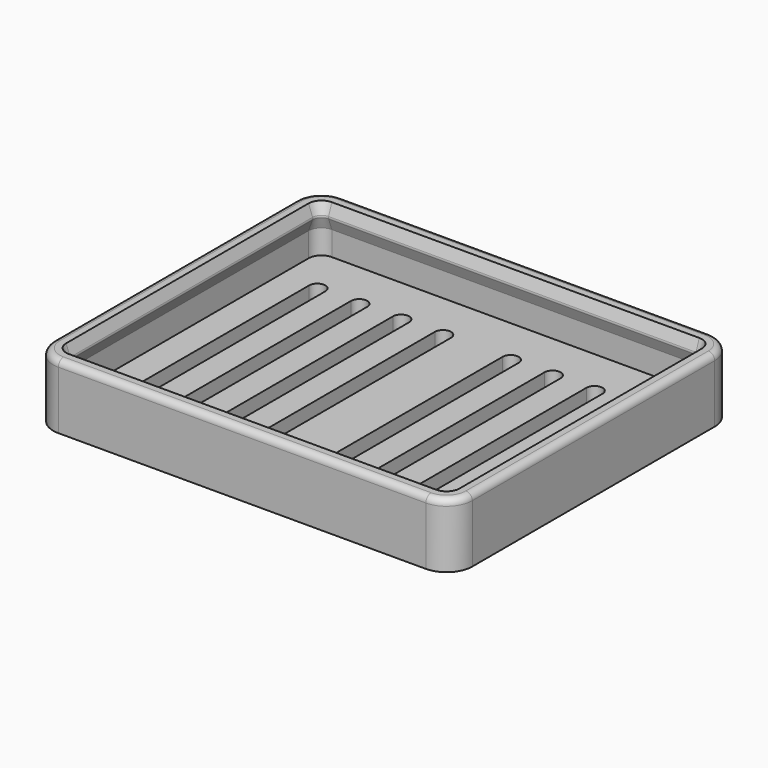
from build123d import *

# Parameters (mm, degrees)
F0_W     = 65
F0_H     = 55
F0_W_2   = 61
F0_H_2   = 51
F1_DEPTH = 2.5
F2_DEPTH = 10
F3_R     = 2
F4_R     = 4
F7_R     = 1


with BuildPart() as f1:
    # F0 (on Top) → F1 (new body)
    with BuildSketch(Plane.XY):
        Rectangle(F0_W, F0_H)
        Rectangle(F0_W_2, F0_H_2, mode=Mode.SUBTRACT)
        Rectangle(F0_W_2, F0_H_2)
        with BuildLine():
            ThreePointArc((-26, 18), (-24.75, 19.25), (-23.5, 18))
            Line((-23.5, 18), (-23.5, -18))
            ThreePointArc((-23.5, -18), (-24.75, -19.25), (-26, -18))
            Line((-26, -18), (-26, 18))
        make_face(mode=Mode.SUBTRACT)
        with BuildLine():
            Line((-19.5, -18), (-19.5, 18))
            ThreePointArc((-19.5, 18), (-18.25, 19.25), (-17, 18))
            Line((-17, 18), (-17, -18))
            ThreePointArc((-17, -18), (-18.25, -19.25), (-19.5, -18))
        make_face(mode=Mode.SUBTRACT)
        with BuildLine():
            Line((-13, -18), (-13, 18))
            ThreePointArc((-13, 18), (-11.75, 19.25), (-10.5, 18))
            Line((-10.5, 18), (-10.5, -18))
            ThreePointArc((-10.5, -18), (-11.75, -19.25), (-13, -18))
        make_face(mode=Mode.SUBTRACT)
        with BuildLine():
            Line((-6.5, -18), (-6.5, 18))
            ThreePointArc((-6.5, 18), (-5.25, 19.25), (-4, 18))
            Line((-4, 18), (-4, -18))
            ThreePointArc((-4, -18), (-5.25, -19.25), (-6.5, -18))
        make_face(mode=Mode.SUBTRACT)
        with BuildLine():
            Line((4, -18), (4, 18))
            ThreePointArc((4, 18), (5.25, 19.25), (6.5, 18))
            Line((6.5, 18), (6.5, -18))
            ThreePointArc((6.5, -18), (5.25, -19.25), (4, -18))
        make_face(mode=Mode.SUBTRACT)
        with BuildLine():
            Line((10.5, -18), (10.5, 18))
            ThreePointArc((10.5, 18), (11.75, 19.25), (13, 18))
            Line((13, 18), (13, -18))
            ThreePointArc((13, -18), (11.75, -19.25), (10.5, -18))
        make_face(mode=Mode.SUBTRACT)
        with BuildLine():
            ThreePointArc((17, 18), (18.25, 19.25), (19.5, 18))
            Line((19.5, 18), (19.5, -18))
            ThreePointArc((19.5, -18), (18.25, -19.25), (17, -18))
            Line((17, -18), (17, 18))
        make_face(mode=Mode.SUBTRACT)
        with BuildLine():
            Line((23.5, -18), (23.5, 18))
            ThreePointArc((23.5, 18), (24.75, 19.25), (26, 18))
            Line((26, 18), (26, -18))
            ThreePointArc((26, -18), (24.75, -19.25), (23.5, -18))
        make_face(mode=Mode.SUBTRACT)
    extrude(amount=F1_DEPTH)

    # F0 (on Top) → F2 (join)
    with BuildSketch(Plane.XY):
        Rectangle(F0_W, F0_H)
        Rectangle(F0_W_2, F0_H_2, mode=Mode.SUBTRACT)
    extrude(amount=F2_DEPTH)

    # F3
    f3_edges = [f1.edges().sort_by_distance(p)[0] for p in [
        (-30.5, 25.5, 6.25),
        (30.5, 25.5, 6.25),
        (-30.5, -25.5, 6.25),
        (30.5, -25.5, 6.25),
    ]]
    fillet(f3_edges, radius=F3_R)

    # F4
    f4_edges = [f1.edges().sort_by_distance(p)[0] for p in [
        (-32.5, 27.5, 5),
        (32.5, 27.5, 5),
        (-32.5, -27.5, 5),
        (32.5, -27.5, 5),
    ]]
    fillet(f4_edges, radius=F4_R)

    # F6: sweep along a path in F6_path
    with BuildLine(Plane(origin=(-30.5, 23.5, 10), x_dir=(0, 1, 0), z_dir=(0, 0, 1))) as f6_path:
        Line((0, 0), (-47, 0))
        ThreePointArc((-47, 0), (-48.4142135624, -0.5857864376), (-49, -2))
        Line((-49, -2), (-49, -59))
        ThreePointArc((-49, -59), (-48.4142135624, -60.4142135624), (-47, -61))
        Line((-47, -61), (0, -61))
        ThreePointArc((0, -61), (1.4142135624, -60.4142135624), (2, -59))
        Line((2, -59), (2, -2))
        ThreePointArc((2, -2), (1.4142135624, -0.5857864376), (0, 0))
    # F5 (on Front) → F6 (sweep)
    with BuildSketch(Plane.XZ):
        with BuildLine():
            Line((-30.5, 10), (-30.5, 6.2521283853))
            Line((-30.5, 6.2521283853), (-29.8801235899, 7.9552248249))
            ThreePointArc((-29.8801235899, 7.9552248249), (-29.85, 8.1260641927), (-29.8801235899, 8.2969035604))
            Line((-29.8801235899, 8.2969035604), (-30.5, 10))
        make_face()
    sweep(path=f6_path.line)

    # F7
    f7_edges = [f1.edges().sort_by_distance(p)[0] for p in [
        (0, 27.5, 10),
    ]]
    fillet(f7_edges, radius=F7_R)


solid = f1.part
